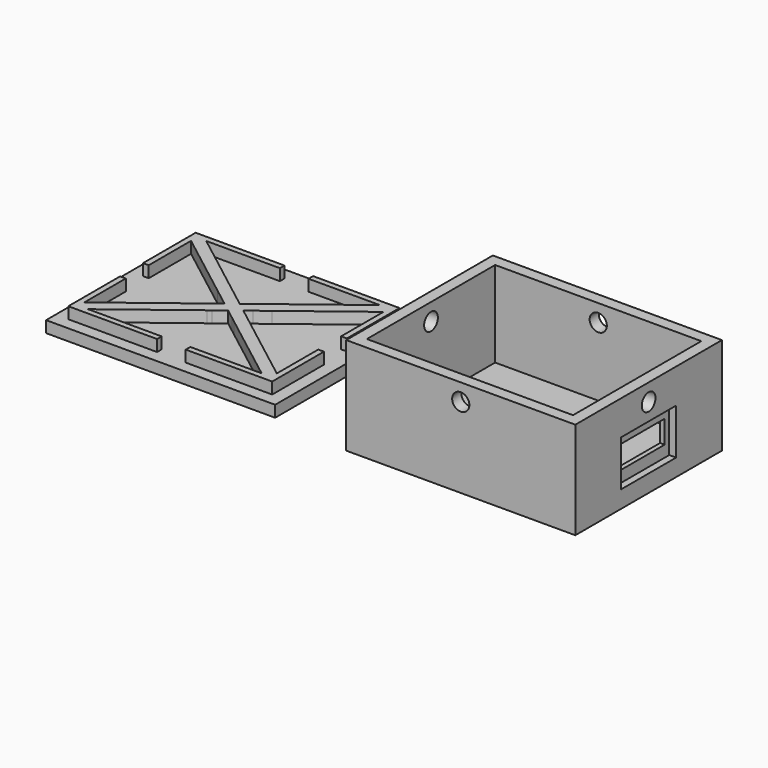
from build123d import *

# Parameters (mm, degrees)
F0_W      = 40
F0_H      = 32
F1_DEPTH  = 17
F2_W      = 36
F2_H      = 28
F3_DEPTH  = 15
F4_R      = 1.5
F5_DEPTH  = 40.001
F6_R      = 1.5
F7_DEPTH  = 32.001
F4_W      = 10
F4_H      = 4
F8_DEPTH  = 2
F9_W      = 40
F9_H      = 32
F10_DEPTH = 2
F12_DEPTH = 2
F4_W_2    = 12
F4_H_2    = 8
F13_DEPTH = 1.2


with BuildPart() as f1:
    # F0 (on Top) → F1 (new body)
    with BuildSketch(Plane.XY):
        with Locations((20, 16)):
            Rectangle(F0_W, F0_H)
    extrude(amount=F1_DEPTH)

    # F2 (on face) → F3 (cut)
    with BuildSketch(Plane.XY.offset(17)):
        with Locations((20, 16)):
            Rectangle(F2_W, F2_H)
    extrude(amount=-F3_DEPTH, mode=Mode.SUBTRACT)

    # F4 (on face) → F5 (cut, through all)
    with BuildSketch(Plane.YZ.offset(40)):
        with Locations((16, 14)):
            Circle(F4_R)
    extrude(amount=-F5_DEPTH, mode=Mode.SUBTRACT)

    # F6 (on face) → F7 (cut, through all)
    with BuildSketch(Plane(origin=(0, 32, 0), x_dir=(-1, 0, 0), z_dir=(0, 1, 0))):
        with Locations((-20, 14)):
            Circle(F6_R)
    extrude(amount=-F7_DEPTH, mode=Mode.SUBTRACT)

    # F4 (on face) → F8 (cut, through all)
    with BuildSketch(Plane.YZ.offset(40)):
        with Locations((16, 7)):
            Rectangle(F4_W, F4_H)
    extrude(amount=-F8_DEPTH, mode=Mode.SUBTRACT)

    # F4 (on face) → F13 (cut)
    with BuildSketch(Plane.YZ.offset(40)):
        with Locations((16, 7)):
            Rectangle(F4_W_2, F4_H_2)
        with Locations((16, 7)):
            Rectangle(F4_W, F4_H, mode=Mode.SUBTRACT)
    extrude(amount=-F13_DEPTH, mode=Mode.SUBTRACT)


with BuildPart() as f10:
    # F9 (on Top) → F10 (new body)
    with BuildSketch(Plane.XY):
        with Locations((-33.6390890081, 17.5289876275)):
            Rectangle(F9_W, F9_H)
    extrude(amount=F10_DEPTH)

    # F11 (on face) → F12 (join)
    with BuildSketch(Plane.XY.offset(2)):
        Polygon((-35.9390890081, 31.4289876275), (-51.4390890081, 31.4289876275), (-51.4390890081, 19.9289876275), (-50.4390890081, 19.9289876275), (-50.4390890081, 29.1681924055), (-50.4390890081, 30.4289876275), (-48.7971231376, 30.4289876275), (-35.9390890081, 30.4289876275), align=None)
        Polygon((-15.8390890081, 31.4289876275), (-30.9390890081, 31.4289876275), (-30.9390890081, 30.4289876275), (-18.4810548786, 30.4289876275), (-16.8390890081, 30.4289876275), (-16.8390890081, 29.1681924055), (-16.8390890081, 19.9289876275), (-15.8390890081, 19.9289876275), align=None)
        Polygon((-50.4390890081, 30.4289876275), (-50.4390890081, 29.1681924055), (-38.406636274, 19.9289876275), (-36.7646704035, 19.9289876275), align=None)
        Polygon((-35.9390890081, 20.5558542781), (-48.7971231376, 30.4289876275), (-50.4390890081, 30.4289876275), (-36.7646704035, 19.9289876275), (-35.9390890081, 19.9289876275), align=None)
        Polygon((-32.8181060728, 18.1593852385), (-33.6390890081, 18.7897828495), (-34.4600719434, 18.1593852385), (-33.6390890081, 17.5289876275), align=None)
        Polygon((-31.9971231376, 17.5289876275), (-32.8181060728, 18.1593852385), (-33.6390890081, 17.5289876275), (-32.8181060728, 16.8985900165), align=None)
        Polygon((-34.4600719434, 18.1593852385), (-35.2810548786, 17.5289876275), (-34.4600719434, 16.8985900165), (-33.6390890081, 17.5289876275), align=None)
        Polygon((-33.6390890081, 17.5289876275), (-34.4600719434, 16.8985900165), (-33.6390890081, 16.2681924055), (-32.8181060728, 16.8985900165), align=None)
        Polygon((-30.9390890081, 18.3414066912), (-30.9390890081, 19.6022019132), (-32.8181060728, 18.1593852385), (-31.9971231376, 17.5289876275), align=None)
        Polygon((-30.9390890081, 19.9289876275), (-32.1554734833, 19.9289876275), (-33.6390890081, 18.7897828495), (-32.8181060728, 18.1593852385), (-30.9390890081, 19.6022019132), align=None)
        Polygon((-35.2810548786, 17.5289876275), (-35.9390890081, 17.0237114209), (-35.9390890081, 15.7629161989), (-34.4600719434, 16.8985900165), align=None)
        Polygon((-34.4600719434, 16.8985900165), (-35.9390890081, 15.7629161989), (-35.9390890081, 14.9289876275), (-35.3831696492, 14.9289876275), (-33.6390890081, 16.2681924055), align=None)
        Polygon((-30.9390890081, 14.1949781198), (-18.4810548786, 4.6289876275), (-16.8390890081, 4.6289876275), (-30.2530424965, 14.9289876275), (-30.9390890081, 14.9289876275), align=None)
        Polygon((-16.8390890081, 4.6289876275), (-16.8390890081, 5.8897828495), (-28.611076626, 14.9289876275), (-30.2530424965, 14.9289876275), align=None)
        Polygon((-35.9390890081, 17.0237114209), (-38.6671013903, 14.9289876275), (-37.0251355197, 14.9289876275), (-35.9390890081, 15.7629161989), align=None)
        Polygon((-36.7646704035, 19.9289876275), (-38.406636274, 19.9289876275), (-35.9390890081, 18.034263834), (-35.9390890081, 19.295059056), align=None)
        Polygon((-35.9390890081, 19.295059056), (-35.9390890081, 18.034263834), (-35.2810548786, 17.5289876275), (-34.4600719434, 18.1593852385), align=None)
        Polygon((-33.6390890081, 18.7897828495), (-35.1227045329, 19.9289876275), (-35.9390890081, 19.9289876275), (-35.9390890081, 19.295059056), (-34.4600719434, 18.1593852385), align=None)
        Polygon((-35.1227045329, 19.9289876275), (-35.9390890081, 20.5558542781), (-35.9390890081, 19.9289876275), align=None)
        Polygon((-35.9390890081, 15.7629161989), (-37.0251355197, 14.9289876275), (-35.9390890081, 14.9289876275), align=None)
        Polygon((-32.8181060728, 16.8985900165), (-33.6390890081, 16.2681924055), (-31.895008367, 14.9289876275), (-30.9390890081, 14.9289876275), (-30.9390890081, 15.4557733418), align=None)
        Polygon((-30.9390890081, 16.7165685638), (-31.9971231376, 17.5289876275), (-32.8181060728, 16.8985900165), (-30.9390890081, 15.4557733418), align=None)
        Polygon((-30.2530424965, 14.9289876275), (-28.611076626, 14.9289876275), (-30.9390890081, 16.7165685638), (-30.9390890081, 15.4557733418), align=None)
        Polygon((-30.9390890081, 14.9289876275), (-30.2530424965, 14.9289876275), (-30.9390890081, 15.4557733418), align=None)
        Polygon((-31.895008367, 14.9289876275), (-30.9390890081, 14.1949781198), (-30.9390890081, 14.9289876275), align=None)
        Polygon((-35.9390890081, 19.295059056), (-35.9390890081, 19.9289876275), (-36.7646704035, 19.9289876275), align=None)
        Polygon((-30.9390890081, 18.3414066912), (-28.8715417422, 19.9289876275), (-30.5135076128, 19.9289876275), (-30.9390890081, 19.6022019132), align=None)
        Polygon((-30.5135076128, 19.9289876275), (-30.9390890081, 19.9289876275), (-30.9390890081, 19.6022019132), align=None)
        Polygon((-30.9390890081, 19.9289876275), (-30.9390890081, 20.8629971352), (-32.1554734833, 19.9289876275), align=None)
        Polygon((-16.8390890081, 30.4289876275), (-18.4810548786, 30.4289876275), (-30.9390890081, 20.8629971352), (-30.9390890081, 19.9289876275), (-30.5135076128, 19.9289876275), align=None)
        Polygon((-16.8390890081, 29.1681924055), (-16.8390890081, 30.4289876275), (-30.5135076128, 19.9289876275), (-28.8715417422, 19.9289876275), align=None)
        Polygon((-37.0251355197, 14.9289876275), (-50.4390890081, 4.6289876275), (-48.7971231376, 4.6289876275), (-35.9390890081, 14.5021209769), (-35.9390890081, 14.9289876275), align=None)
        Polygon((-38.6671013903, 14.9289876275), (-50.4390890081, 5.8897828495), (-50.4390890081, 4.6289876275), (-37.0251355197, 14.9289876275), align=None)
        Polygon((-50.4390890081, 14.9289876275), (-51.4390890081, 14.9289876275), (-51.4390890081, 3.6289876275), (-35.9390890081, 3.6289876275), (-35.9390890081, 4.6289876275), (-48.7971231376, 4.6289876275), (-50.4390890081, 4.6289876275), (-50.4390890081, 5.8897828495), align=None)
        Polygon((-15.8390890081, 3.6289876275), (-15.8390890081, 14.9289876275), (-16.8390890081, 14.9289876275), (-16.8390890081, 5.8897828495), (-16.8390890081, 4.6289876275), (-18.4810548786, 4.6289876275), (-30.9390890081, 4.6289876275), (-30.9390890081, 3.6289876275), align=None)
        Polygon((-35.9390890081, 14.9289876275), (-35.9390890081, 14.5021209769), (-35.3831696492, 14.9289876275), align=None)
    extrude(amount=F12_DEPTH)


solid = Compound([f1.part, f10.part])
